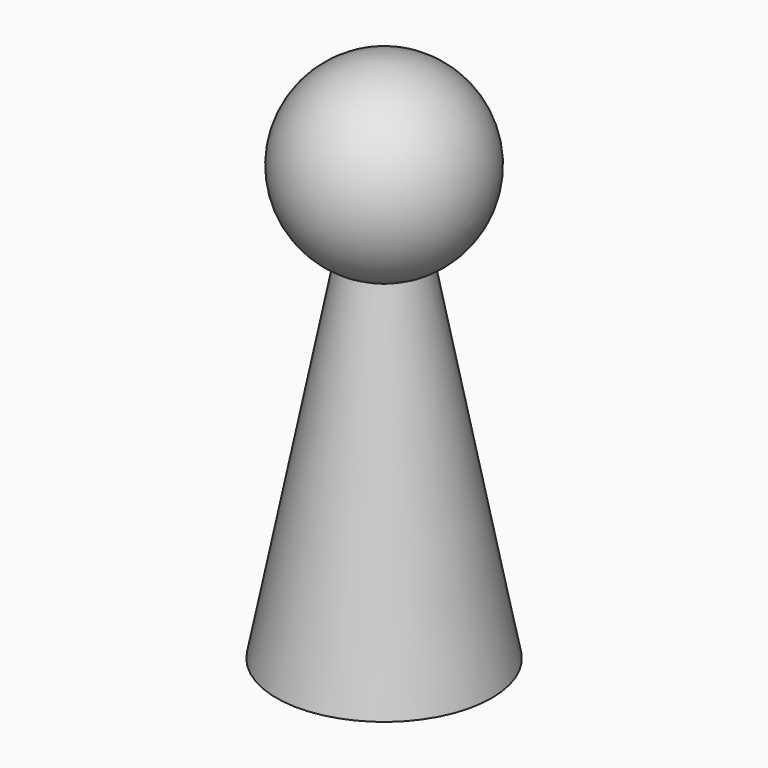
from build123d import *


# Not quite as in the source:
# - a feature names something its author has since deleted; it is built from what else it names


with BuildPart() as f1:
    # F0 (on Front) → F1 (revolve)
    with BuildSketch(Plane.XZ):
        with BuildLine():
            Line((21.2230402976, -44.6271188557), (7.7761935474, 24.4178486332))
            ThreePointArc((7.7761935474, 24.4178486332), (17.8766324697, 44.9836060593), (0, 59.3152234305))
            Line((0, 59.3152234305), (0, 22.6850768577))
            Line((0, 22.6850768577), (0, -43.8756793737))
            Line((0, -43.8756793737), (21.2230402976, -44.6271188557))
        make_face()
    revolve(axis=Axis((0, 0, -10.595301258), (0, 0, -1)))


solid = f1.part
